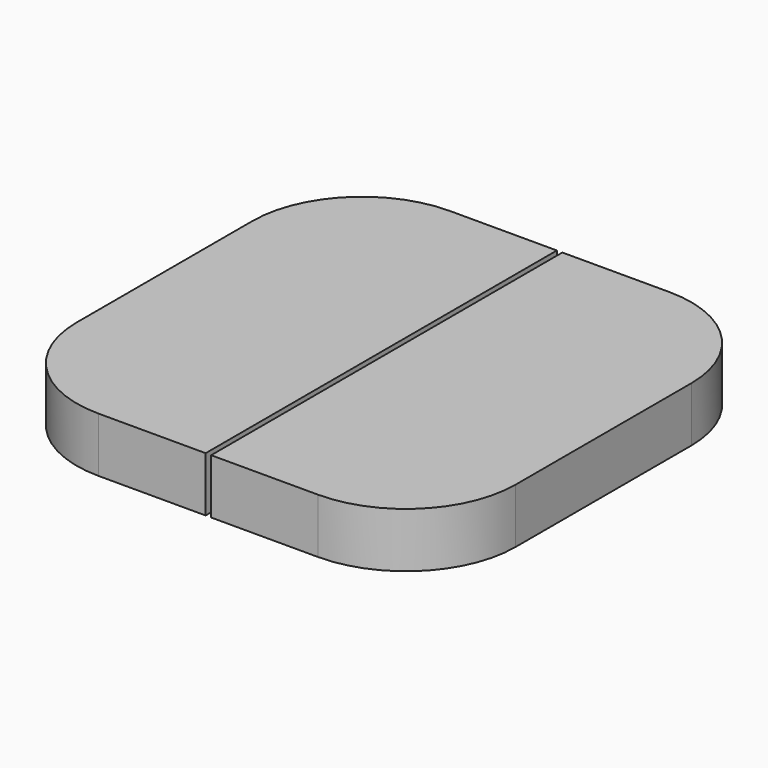
from build123d import *

# Parameters (mm, degrees)
F0_R     = 25.4
F1_DEPTH = 25.4


# Not quite as in the source:
# - the program builds the solid bodies; features that only make, move or delete a surface that nothing else refers to are left out


with BuildPart() as f1:
    # F0 (on Top) → F1 (new body)
    with BuildSketch(Plane.XY):
        with BuildLine():
            Line((-66.6004060161, 166.1117917925), (-116.1304060161, 166.1117917925))
            ThreePointArc((-116.1304060161, 166.1117917925), (-152.0514305004, 151.2328162768), (-166.9304060161, 115.3117917925))
            Line((-166.9304060161, 115.3117917925), (-166.9304060161, 13.7117917925))
            ThreePointArc((-166.9304060161, 13.7117917925), (-152.0514305004, -22.2092326918), (-116.1304060161, -37.0882082075))
            Line((-116.1304060161, -37.0882082075), (-66.6004060161, -37.0882082075))
            Line((-66.6004060161, -37.0882082075), (-66.6004060161, 166.1117917925))
        make_face()
        with Locations((-116.1304060161, 115.3117917925)):
            Circle(F0_R, mode=Mode.SUBTRACT)
        with Locations((-116.1304060161, 115.3117917925)):
            Circle(F0_R)
    extrude(amount=F1_DEPTH)


with BuildPart() as f1b:
    # F0 (on Top) → F1, piece 2 (new body)
    with BuildSketch(Plane.XY):
        with BuildLine():
            Line((-14.5304060161, 166.1117917925), (-64.0604060161, 166.1117917925))
            Line((-64.0604060161, 166.1117917925), (-64.0604060161, -37.0882082075))
            Line((-64.0604060161, -37.0882082075), (-14.5304060161, -37.0882082075))
            ThreePointArc((-14.5304060161, -37.0882082075), (21.3906184682, -22.2092326918), (36.2695939839, 13.7117917925))
            Line((36.2695939839, 13.7117917925), (36.2695939839, 115.3117917925))
            ThreePointArc((36.2695939839, 115.3117917925), (21.3906184682, 151.2328162768), (-14.5304060161, 166.1117917925))
        make_face()
        with Locations((-14.5304060161, 13.7117917925)):
            Circle(F0_R, mode=Mode.SUBTRACT)
        with Locations((-14.5304060161, 13.7117917925)):
            Circle(F0_R)
    extrude(amount=F1_DEPTH)


solid = Compound([f1.part, f1b.part])
